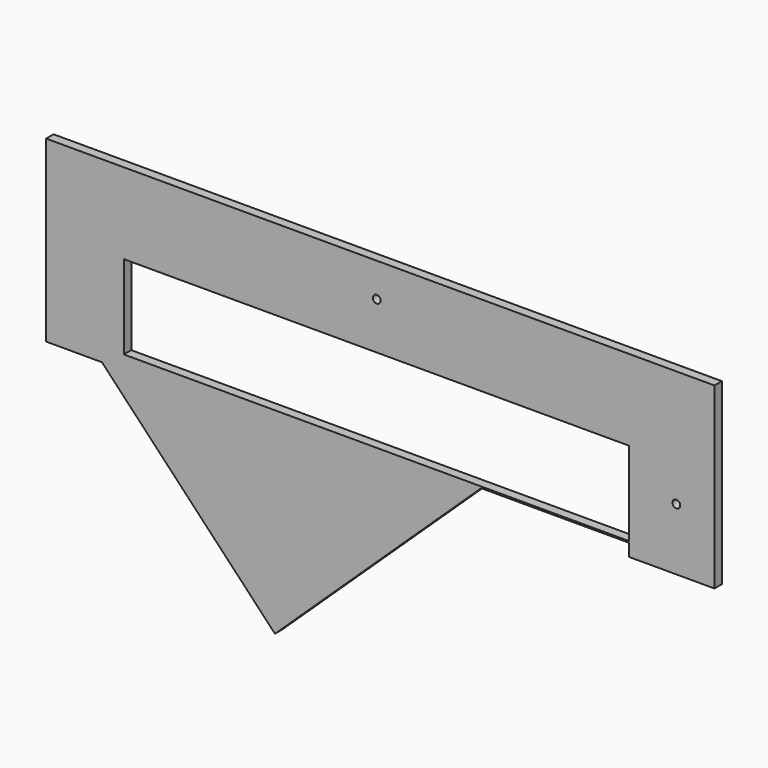
from build123d import *

# Parameters (mm, degrees)
F0_W     = 325
F0_H     = 54
F0_R     = 2.5
F1_DEPTH = 6


# Not quite as in the source:
# - a feature names something its author has since deleted; it is built from what else it names


with BuildPart() as f1:
    # F0 (on Front) → F1 (new body)
    with BuildSketch(Plane.XZ):
        Polygon((0, 115), (0, 0), (35.9275913919, 0), (50, 0), (50, 8), (279.8869819123, 8), (375, 8), (375, 0), (430, 0), (430, 115), align=None)
        with Locations((212.5, 36)):
            Rectangle(F0_W, F0_H, mode=Mode.SUBTRACT)
        with Locations((212.7146603412, 93.1771022268)):
            Circle(F0_R, mode=Mode.SUBTRACT)
        with Locations((405.4770870114, 39.8606238714)):
            Circle(F0_R, mode=Mode.SUBTRACT)
        Polygon((50, 0), (35.9275913919, 0), (147.2313553095, -117.5774261355), (279.8869819123, 8), (50, 8), align=None)
    extrude(amount=F1_DEPTH)


solid = f1.part
